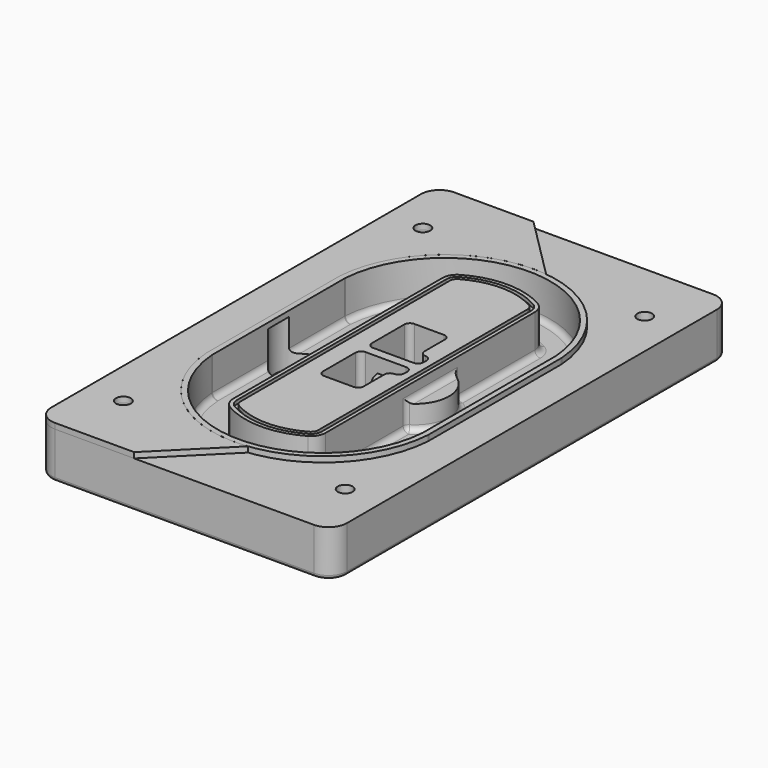
from build123d import *

# Parameters (mm, degrees)
F0_R      = 4
F1_DEPTH  = 25
F2_DEPTH  = 3
F3_DEPTH  = 18
F5_DEPTH  = 21
F6_DEPTH  = 2
F8_DEPTH  = 20
F9_DEPTH  = 16
F10_DEPTH = 25
F7_R      = 6
F7_R_2    = 4
F11_DEPTH = 6
F13_DEPTH = 9
F14_R     = 3
F15_R     = 2
F16_R     = 4
F17_DEPTH = 3


with BuildPart() as f1:
    # F0 (on Top) → F1 (new body)
    with BuildSketch(Plane.XY):
        with BuildLine():
            ThreePointArc((-80, -125), (-77.0710678119, -132.0710678119), (-70, -135))
            Line((-70, -135), (70, -135))
            ThreePointArc((70, -135), (77.0710678119, -132.0710678119), (80, -125))
            Line((80, -125), (80, 125))
            ThreePointArc((80, 125), (77.0710678119, 132.0710678119), (70, 135))
            Line((70, 135), (-70, 135))
            ThreePointArc((-70, 135), (-77.0710678119, 132.0710678119), (-80, 125))
            Line((-80, 125), (-80, -125))
        make_face()
        with Locations((-60, -101.25)):
            Circle(F0_R, mode=Mode.SUBTRACT)
        with Locations((60, -101.25)):
            Circle(F0_R, mode=Mode.SUBTRACT)
        with Locations((-60, 101.25)):
            Circle(F0_R, mode=Mode.SUBTRACT)
        with BuildLine():
            ThreePointArc((-64, 44.6627429245), (-63.991269098, 45.1571001106), (-63.9650872818, 45.650840699))
            ThreePointArc((-63.9650872818, 45.650840699), (0, 105.25), (63.9650872818, 45.650840699))
            ThreePointArc((63.9650872818, 45.650840699), (63.991269098, 45.1571001106), (64, 44.6627429245))
            Line((64, 44.6627429245), (64, -44.6627429245))
            ThreePointArc((64, -44.6627429245), (63.991269098, -45.1571001106), (63.9650872818, -45.650840699))
            ThreePointArc((63.9650872818, -45.650840699), (0, -105.25), (-63.9650872818, -45.650840699))
            ThreePointArc((-63.9650872818, -45.650840699), (-63.991269098, -45.1571001106), (-64, -44.6627429245))
            Line((-64, -44.6627429245), (-64, 44.6627429245))
        make_face(mode=Mode.SUBTRACT)
        with Locations((60, 101.25)):
            Circle(F0_R, mode=Mode.SUBTRACT)
        with BuildLine():
            ThreePointArc((63.9650872818, 45.650840699), (0, 105.25), (-63.9650872818, 45.650840699))
            ThreePointArc((-63.9650872818, 45.650840699), (-63.991269098, 45.1571001106), (-64, 44.6627429245))
            Line((-64, 44.6627429245), (-64, -44.6627429245))
            ThreePointArc((-64, -44.6627429245), (-63.991269098, -45.1571001106), (-63.9650872818, -45.650840699))
            ThreePointArc((-63.9650872818, -45.650840699), (0, -105.25), (63.9650872818, -45.650840699))
            ThreePointArc((63.9650872818, -45.650840699), (63.991269098, -45.1571001106), (64, -44.6627429245))
            Line((64, -44.6627429245), (64, 44.6627429245))
            ThreePointArc((64, 44.6627429245), (63.991269098, 45.1571001106), (63.9650872818, 45.650840699))
        make_face()
        with BuildLine():
            Line((-60, -44.6627429245), (-60, 44.6627429245))
            ThreePointArc((-60, 44.6627429245), (-59.9937636414, 45.0158552003), (-59.9750623441, 45.3685270491))
            ThreePointArc((-59.9750623441, 45.3685270491), (0, 101.25), (59.9750623441, 45.3685270491))
            ThreePointArc((59.9750623441, 45.3685270491), (59.9937636414, 45.0158552003), (60, 44.6627429245))
            Line((60, 44.6627429245), (60, -44.6627429245))
            ThreePointArc((60, -44.6627429245), (59.9937636414, -45.0158552003), (59.9750623441, -45.3685270491))
            ThreePointArc((59.9750623441, -45.3685270491), (0, -101.25), (-59.9750623441, -45.3685270491))
            ThreePointArc((-59.9750623441, -45.3685270491), (-59.9937636414, -45.0158552003), (-60, -44.6627429245))
        make_face(mode=Mode.SUBTRACT)
        with BuildLine():
            ThreePointArc((-59.9750623441, 45.3685270491), (-59.9937636414, 45.0158552003), (-60, 44.6627429245))
            Line((-60, 44.6627429245), (-60, -44.6627429245))
            ThreePointArc((-60, -44.6627429245), (-59.9937636414, -45.0158552003), (-59.9750623441, -45.3685270491))
            ThreePointArc((-59.9750623441, -45.3685270491), (0, -101.25), (59.9750623441, -45.3685270491))
            ThreePointArc((59.9750623441, -45.3685270491), (59.9937636414, -45.0158552003), (60, -44.6627429245))
            Line((60, -44.6627429245), (60, 44.6627429245))
            ThreePointArc((60, 44.6627429245), (59.9937636414, 45.0158552003), (59.9750623441, 45.3685270491))
            ThreePointArc((59.9750623441, 45.3685270491), (0, 101.25), (-59.9750623441, 45.3685270491))
        make_face()
        with BuildLine():
            ThreePointArc((56.9825436409, 45.1567918117), (56.995634549, 44.9099215176), (57, 44.6627429245))
            Line((57, 44.6627429245), (57, -44.6627429245))
            ThreePointArc((57, -44.6627429245), (56.995634549, -44.9099215176), (56.9825436409, -45.1567918117))
            ThreePointArc((56.9825436409, -45.1567918117), (0, -98.25), (-56.9825436409, -45.1567918117))
            ThreePointArc((-56.9825436409, -45.1567918117), (-56.995634549, -44.9099215176), (-57, -44.6627429245))
            Line((-57, -44.6627429245), (-57, 44.6627429245))
            ThreePointArc((-57, 44.6627429245), (-56.995634549, 44.9099215176), (-56.9825436409, 45.1567918117))
            ThreePointArc((-56.9825436409, 45.1567918117), (0, 98.25), (56.9825436409, 45.1567918117))
        make_face(mode=Mode.SUBTRACT)
        with BuildLine():
            Line((57, -44.6627429245), (57, 44.6627429245))
            ThreePointArc((57, 44.6627429245), (56.995634549, 44.9099215176), (56.9825436409, 45.1567918117))
            ThreePointArc((56.9825436409, 45.1567918117), (0, 98.25), (-56.9825436409, 45.1567918117))
            ThreePointArc((-56.9825436409, 45.1567918117), (-56.995634549, 44.9099215176), (-57, 44.6627429245))
            Line((-57, 44.6627429245), (-57, -44.6627429245))
            ThreePointArc((-57, -44.6627429245), (-56.995634549, -44.9099215176), (-56.9825436409, -45.1567918117))
            ThreePointArc((-56.9825436409, -45.1567918117), (0, -98.25), (56.9825436409, -45.1567918117))
            ThreePointArc((56.9825436409, -45.1567918117), (56.995634549, -44.9099215176), (57, -44.6627429245))
        make_face()
    extrude(amount=-F1_DEPTH)

    # F0 (on Top) → F2 (join)
    with BuildSketch(Plane.XY):
        with BuildLine():
            ThreePointArc((-59.9750623441, 45.3685270491), (-59.9937636414, 45.0158552003), (-60, 44.6627429245))
            Line((-60, 44.6627429245), (-60, -44.6627429245))
            ThreePointArc((-60, -44.6627429245), (-59.9937636414, -45.0158552003), (-59.9750623441, -45.3685270491))
            ThreePointArc((-59.9750623441, -45.3685270491), (0, -101.25), (59.9750623441, -45.3685270491))
            ThreePointArc((59.9750623441, -45.3685270491), (59.9937636414, -45.0158552003), (60, -44.6627429245))
            Line((60, -44.6627429245), (60, 44.6627429245))
            ThreePointArc((60, 44.6627429245), (59.9937636414, 45.0158552003), (59.9750623441, 45.3685270491))
            ThreePointArc((59.9750623441, 45.3685270491), (0, 101.25), (-59.9750623441, 45.3685270491))
        make_face()
        with BuildLine():
            ThreePointArc((56.9825436409, 45.1567918117), (56.995634549, 44.9099215176), (57, 44.6627429245))
            Line((57, 44.6627429245), (57, -44.6627429245))
            ThreePointArc((57, -44.6627429245), (56.995634549, -44.9099215176), (56.9825436409, -45.1567918117))
            ThreePointArc((56.9825436409, -45.1567918117), (0, -98.25), (-56.9825436409, -45.1567918117))
            ThreePointArc((-56.9825436409, -45.1567918117), (-56.995634549, -44.9099215176), (-57, -44.6627429245))
            Line((-57, -44.6627429245), (-57, 44.6627429245))
            ThreePointArc((-57, 44.6627429245), (-56.995634549, 44.9099215176), (-56.9825436409, 45.1567918117))
            ThreePointArc((-56.9825436409, 45.1567918117), (0, 98.25), (56.9825436409, 45.1567918117))
        make_face(mode=Mode.SUBTRACT)
    extrude(amount=F2_DEPTH)

    # F0 (on Top) → F3 (cut)
    with BuildSketch(Plane.XY):
        with BuildLine():
            Line((57, -44.6627429245), (57, 44.6627429245))
            ThreePointArc((57, 44.6627429245), (56.995634549, 44.9099215176), (56.9825436409, 45.1567918117))
            ThreePointArc((56.9825436409, 45.1567918117), (0, 98.25), (-56.9825436409, 45.1567918117))
            ThreePointArc((-56.9825436409, 45.1567918117), (-56.995634549, 44.9099215176), (-57, 44.6627429245))
            Line((-57, 44.6627429245), (-57, -44.6627429245))
            ThreePointArc((-57, -44.6627429245), (-56.995634549, -44.9099215176), (-56.9825436409, -45.1567918117))
            ThreePointArc((-56.9825436409, -45.1567918117), (0, -98.25), (56.9825436409, -45.1567918117))
            ThreePointArc((56.9825436409, -45.1567918117), (56.995634549, -44.9099215176), (57, -44.6627429245))
        make_face()
    extrude(amount=-F3_DEPTH, mode=Mode.SUBTRACT)

    # F4 (on face) → F5 (join, through all)
    with BuildSketch(Plane.XY.offset(3)):
        with BuildLine():
            ThreePointArc((-25, -70.7141132851), (-23.9239722661, -74.7214325959), (-20.9853479853, -77.6507552274))
            ThreePointArc((-20.9853479853, -77.6507552274), (0, -83.25), (20.9853479853, -77.6507552274))
            ThreePointArc((20.9853479853, -77.6507552274), (23.9239722661, -74.7214325959), (25, -70.7141132851))
            Line((25, -70.7141132851), (25, 70.7141132851))
            ThreePointArc((25, 70.7141132851), (23.9239722661, 74.7214325959), (20.9853479853, 77.6507552274))
            ThreePointArc((20.9853479853, 77.6507552274), (0, 83.25), (-20.9853479853, 77.6507552274))
            ThreePointArc((-20.9853479853, 77.6507552274), (-23.9239722661, 74.7214325959), (-25, 70.7141132851))
            Line((-25, 70.7141132851), (-25, -70.7141132851))
        make_face()
        with BuildLine():
            ThreePointArc((19.989010989, 75.9165947419), (22.1929791996, 73.7196027682), (23, 70.7141132851))
            Line((23, 70.7141132851), (23, -70.7141132851))
            ThreePointArc((23, -70.7141132851), (22.1929791996, -73.7196027682), (19.989010989, -75.9165947419))
            ThreePointArc((19.989010989, -75.9165947419), (0, -81.25), (-19.989010989, -75.9165947419))
            ThreePointArc((-19.989010989, -75.9165947419), (-22.1929791996, -73.7196027682), (-23, -70.7141132851))
            Line((-23, -70.7141132851), (-23, 70.7141132851))
            ThreePointArc((-23, 70.7141132851), (-22.1929791996, 73.7196027682), (-19.989010989, 75.9165947419))
            ThreePointArc((-19.989010989, 75.9165947419), (0, 81.25), (19.989010989, 75.9165947419))
        make_face(mode=Mode.SUBTRACT)
        with BuildLine():
            Line((23, -70.7141132851), (23, 70.7141132851))
            ThreePointArc((23, 70.7141132851), (22.1929791996, 73.7196027682), (19.989010989, 75.9165947419))
            ThreePointArc((19.989010989, 75.9165947419), (0, 81.25), (-19.989010989, 75.9165947419))
            ThreePointArc((-19.989010989, 75.9165947419), (-22.1929791996, 73.7196027682), (-23, 70.7141132851))
            Line((-23, 70.7141132851), (-23, -70.7141132851))
            ThreePointArc((-23, -70.7141132851), (-22.1929791996, -73.7196027682), (-19.989010989, -75.9165947419))
            ThreePointArc((-19.989010989, -75.9165947419), (0, -81.25), (19.989010989, -75.9165947419))
            ThreePointArc((19.989010989, -75.9165947419), (22.1929791996, -73.7196027682), (23, -70.7141132851))
        make_face()
        with BuildLine():
            ThreePointArc((18.9926739927, 74.1824342563), (20.461986133, 72.7177729405), (21, 70.7141132851))
            Line((21, 70.7141132851), (21, -70.7141132851))
            ThreePointArc((21, -70.7141132851), (20.461986133, -72.7177729405), (18.9926739927, -74.1824342563))
            ThreePointArc((18.9926739927, -74.1824342563), (0, -79.25), (-18.9926739927, -74.1824342563))
            ThreePointArc((-18.9926739927, -74.1824342563), (-20.461986133, -72.7177729405), (-21, -70.7141132851))
            Line((-21, -70.7141132851), (-21, 70.7141132851))
            ThreePointArc((-21, 70.7141132851), (-20.461986133, 72.7177729405), (-18.9926739927, 74.1824342563))
            ThreePointArc((-18.9926739927, 74.1824342563), (0, 79.25), (18.9926739927, 74.1824342563))
        make_face(mode=Mode.SUBTRACT)
        with BuildLine():
            Line((21, -70.7141132851), (21, 70.7141132851))
            ThreePointArc((21, 70.7141132851), (20.461986133, 72.7177729405), (18.9926739927, 74.1824342563))
            ThreePointArc((18.9926739927, 74.1824342563), (0, 79.25), (-18.9926739927, 74.1824342563))
            ThreePointArc((-18.9926739927, 74.1824342563), (-20.461986133, 72.7177729405), (-21, 70.7141132851))
            Line((-21, 70.7141132851), (-21, -70.7141132851))
            ThreePointArc((-21, -70.7141132851), (-20.461986133, -72.7177729405), (-18.9926739927, -74.1824342563))
            ThreePointArc((-18.9926739927, -74.1824342563), (0, -79.25), (18.9926739927, -74.1824342563))
            ThreePointArc((18.9926739927, -74.1824342563), (20.461986133, -72.7177729405), (21, -70.7141132851))
        make_face()
        with BuildLine():
            Line((-8, -2.5), (14, -2.5))
            ThreePointArc((14, -2.5), (16.1213203436, -3.3786796564), (17, -5.5))
            Line((17, -5.5), (17, -7.5))
            ThreePointArc((17, -7.5), (16.1213203436, -9.6213203436), (14, -10.5))
            ThreePointArc((14, -10.5), (11.8786796564, -11.3786796564), (11, -13.5))
            Line((11, -13.5), (11, -27.5))
            ThreePointArc((11, -27.5), (10.1213203436, -29.6213203436), (8, -30.5))
            Line((8, -30.5), (-8, -30.5))
            ThreePointArc((-8, -30.5), (-10.1213203436, -29.6213203436), (-11, -27.5))
            Line((-11, -27.5), (-11, -5.5))
            ThreePointArc((-11, -5.5), (-10.1213203436, -3.3786796564), (-8, -2.5))
        make_face(mode=Mode.SUBTRACT)
        with BuildLine():
            ThreePointArc((-8, 2.5), (-10.1213203436, 3.3786796564), (-11, 5.5))
            Line((-11, 5.5), (-11, 27.5))
            ThreePointArc((-11, 27.5), (-10.1213203436, 29.6213203436), (-8, 30.5))
            Line((-8, 30.5), (8, 30.5))
            ThreePointArc((8, 30.5), (10.1213203436, 29.6213203436), (11, 27.5))
            Line((11, 27.5), (11, 13.5))
            ThreePointArc((11, 13.5), (11.8786796564, 11.3786796564), (14, 10.5))
            ThreePointArc((14, 10.5), (16.1213203436, 9.6213203436), (17, 7.5))
            Line((17, 7.5), (17, 5.5))
            ThreePointArc((17, 5.5), (16.1213203436, 3.3786796564), (14, 2.5))
            Line((14, 2.5), (-8, 2.5))
        make_face(mode=Mode.SUBTRACT)
    extrude(amount=-F5_DEPTH)

    # F4 (on face) → F6 (cut)
    with BuildSketch(Plane.XY.offset(3)):
        with BuildLine():
            Line((23, -70.7141132851), (23, 70.7141132851))
            ThreePointArc((23, 70.7141132851), (22.1929791996, 73.7196027682), (19.989010989, 75.9165947419))
            ThreePointArc((19.989010989, 75.9165947419), (0, 81.25), (-19.989010989, 75.9165947419))
            ThreePointArc((-19.989010989, 75.9165947419), (-22.1929791996, 73.7196027682), (-23, 70.7141132851))
            Line((-23, 70.7141132851), (-23, -70.7141132851))
            ThreePointArc((-23, -70.7141132851), (-22.1929791996, -73.7196027682), (-19.989010989, -75.9165947419))
            ThreePointArc((-19.989010989, -75.9165947419), (0, -81.25), (19.989010989, -75.9165947419))
            ThreePointArc((19.989010989, -75.9165947419), (22.1929791996, -73.7196027682), (23, -70.7141132851))
        make_face()
        with BuildLine():
            ThreePointArc((18.9926739927, 74.1824342563), (20.461986133, 72.7177729405), (21, 70.7141132851))
            Line((21, 70.7141132851), (21, -70.7141132851))
            ThreePointArc((21, -70.7141132851), (20.461986133, -72.7177729405), (18.9926739927, -74.1824342563))
            ThreePointArc((18.9926739927, -74.1824342563), (0, -79.25), (-18.9926739927, -74.1824342563))
            ThreePointArc((-18.9926739927, -74.1824342563), (-20.461986133, -72.7177729405), (-21, -70.7141132851))
            Line((-21, -70.7141132851), (-21, 70.7141132851))
            ThreePointArc((-21, 70.7141132851), (-20.461986133, 72.7177729405), (-18.9926739927, 74.1824342563))
            ThreePointArc((-18.9926739927, 74.1824342563), (0, 79.25), (18.9926739927, 74.1824342563))
        make_face(mode=Mode.SUBTRACT)
    extrude(amount=-F6_DEPTH, mode=Mode.SUBTRACT)

    # F7 (on face) → F8 (join)
    with BuildSketch(Plane(origin=(0, 0, -25), x_dir=(1, 0, 0), z_dir=(0, 0, -1))):
        with BuildLine():
            ThreePointArc((3.28842436, 0), (16.7567035675, 13.4682792075), (30.224982775, 0))
            Line((30.224982775, 0), (35.224982775, 0))
            ThreePointArc((35.224982775, 0), (16.7567035675, 18.4682792075), (-1.71157564, 0))
            Line((-1.71157564, 0), (3.28842436, 0))
        make_face()
        with BuildLine():
            Line((3.28842436, 0), (30.224982775, 0))
            ThreePointArc((30.224982775, 0), (16.7567035675, 13.4682792075), (3.28842436, 0))
        make_face()
        with BuildLine():
            ThreePointArc((3.28842436, 0), (16.7567035675, -13.4682792075), (30.224982775, 0))
            Line((30.224982775, 0), (3.28842436, 0))
        make_face()
        with BuildLine():
            Line((35.224982775, 0), (30.224982775, 0))
            ThreePointArc((30.224982775, 0), (16.7567035675, -13.4682792075), (3.28842436, 0))
            Line((3.28842436, 0), (-1.71157564, 0))
            ThreePointArc((-1.71157564, 0), (16.7567035675, -18.4682792075), (35.224982775, 0))
        make_face()
    extrude(amount=-F8_DEPTH)

    # F7 (on face) → F9 (cut)
    with BuildSketch(Plane(origin=(0, 0, -25), x_dir=(1, 0, 0), z_dir=(0, 0, -1))):
        with BuildLine():
            Line((3.28842436, 0), (30.224982775, 0))
            ThreePointArc((30.224982775, 0), (16.7567035675, 13.4682792075), (3.28842436, 0))
        make_face()
        with BuildLine():
            ThreePointArc((3.28842436, 0), (16.7567035675, -13.4682792075), (30.224982775, 0))
            Line((30.224982775, 0), (3.28842436, 0))
        make_face()
    extrude(amount=-F9_DEPTH, mode=Mode.SUBTRACT)

    # F7 (on face) → F10 (cut)
    with BuildSketch(Plane(origin=(0, 0, -25), x_dir=(1, 0, 0), z_dir=(0, 0, -1))):
        with BuildLine():
            Line((-59.0318229325, 0), (-32.0952645175, 0))
            ThreePointArc((-32.0952645175, 0), (-45.563543725, 13.4682792075), (-59.0318229325, 0))
        make_face()
        with BuildLine():
            ThreePointArc((-59.0318229325, 0), (-45.563543725, -13.4682792075), (-32.0952645175, 0))
            Line((-32.0952645175, 0), (-59.0318229325, 0))
        make_face()
    extrude(amount=-F10_DEPTH, mode=Mode.SUBTRACT)

    # F7 (on face) → F11 (cut)
    with BuildSketch(Plane(origin=(0, 0, -25), x_dir=(1, 0, 0), z_dir=(0, 0, -1))):
        with Locations((60, -101.25)):
            Circle(F7_R)
        with Locations((60, -101.25)):
            Circle(F7_R_2, mode=Mode.SUBTRACT)
        with Locations((-60, -101.25)):
            Circle(F7_R)
        with Locations((-60, -101.25)):
            Circle(F7_R_2, mode=Mode.SUBTRACT)
        with Locations((-60, 101.25)):
            Circle(F7_R)
        with Locations((-60, 101.25)):
            Circle(F7_R_2, mode=Mode.SUBTRACT)
        with Locations((60, 101.25)):
            Circle(F7_R)
        with Locations((60, 101.25)):
            Circle(F7_R_2, mode=Mode.SUBTRACT)
    extrude(amount=-F11_DEPTH, mode=Mode.SUBTRACT)

    # F12 (on face) → F13 (cut, through all)
    with BuildSketch(Plane(origin=(0, 0, -9), x_dir=(1, 0, 0), z_dir=(0, 0, -1))):
        with BuildLine():
            Line((11, 13.5), (11, 17.5481537753))
            ThreePointArc((11, 17.5481537753), (2.5696536419, 11.8239143813), (-1.5415842455, 2.5))
            Line((-1.5415842455, 2.5), (3.5224848595, 2.5))
            ThreePointArc((3.5224848595, 2.5), (6.1857188154, 8.3455872281), (11.2536447004, 12.2927168648))
            ThreePointArc((11.2536447004, 12.2927168648), (11.0640958889, 12.8831798879), (11, 13.5))
        make_face()
        with BuildLine():
            ThreePointArc((11.2536447004, -12.2927168648), (6.1857188154, -8.3455872281), (3.5224848595, -2.5))
            Line((3.5224848595, -2.5), (-1.5415842455, -2.5))
            ThreePointArc((-1.5415842455, -2.5), (2.5696536419, -11.8239143813), (11, -17.5481537753))
            Line((11, -17.5481537753), (11, -13.5))
            ThreePointArc((11, -13.5), (11.0640958889, -12.8831798879), (11.2536447004, -12.2927168648))
        make_face()
        with BuildLine():
            ThreePointArc((11.2536447004, 12.2927168648), (6.1857188154, 8.3455872281), (3.5224848595, 2.5))
            Line((3.5224848595, 2.5), (14, 2.5))
            ThreePointArc((14, 2.5), (16.1213203436, 3.3786796564), (17, 5.5))
            Line((17, 5.5), (17, 7.5))
            ThreePointArc((17, 7.5), (16.1213203436, 9.6213203436), (14, 10.5))
            ThreePointArc((14, 10.5), (12.3601599782, 10.9878446101), (11.2536447004, 12.2927168648))
        make_face()
        with BuildLine():
            Line((14, -2.5), (3.5224848595, -2.5))
            ThreePointArc((3.5224848595, -2.5), (6.1857188154, -8.3455872281), (11.2536447004, -12.2927168648))
            ThreePointArc((11.2536447004, -12.2927168648), (12.3601599782, -10.9878446101), (14, -10.5))
            ThreePointArc((14, -10.5), (16.1213203436, -9.6213203436), (17, -7.5))
            Line((17, -7.5), (17, -5.5))
            ThreePointArc((17, -5.5), (16.1213203436, -3.3786796564), (14, -2.5))
        make_face()
    extrude(amount=F13_DEPTH, mode=Mode.SUBTRACT)

    # F14
    f14_edges = [f1.edges().sort_by_distance(p)[0] for p in [
        (-57, -25.888126, -18),
        (-57, 25.888126, -18),
        (25, 0, -5),
        (25, 16.526506, -11.5),
        (25, -16.526506, -11.5),
        (25, -43.62031, -18),
        (35.224983, 0, -18),
        (25, 43.62031, -18),
        (0, -98.25, -18),
        (-56.995635, -44.909922, -18),
        (-56.995635, 44.909922, -18),
        (0, 98.25, -18),
        (56.995635, 44.909922, -18),
        (57, 0, -18),
        (56.995635, -44.909922, -18),
        (-25, 0, -18),
        (-23.923972, 74.721433, -18),
        (-23.923972, -74.721433, -18),
        (0, 83.25, -18),
        (0, -83.25, -18),
        (23.923972, 74.721433, -18),
        (23.923972, -74.721433, -18),
    ]]
    fillet(f14_edges, radius=F14_R)

    # F15
    f15_edges = [f1.edges().sort_by_distance(p)[0] for p in [
        (0, -135, -25),
        (-77.071068, -132.071068, -25),
        (-80, 0, -25),
        (-77.071068, 132.071068, -25),
        (77.071068, -132.071068, -25),
        (0, 135, -25),
        (80, 0, -25),
        (77.071068, 132.071068, -25),
    ]]
    fillet(f15_edges, radius=F15_R)


with BuildPart() as f17:
    # F16 (on face) → F17 (new body, through all)
    with BuildSketch(Plane.XY):
        with BuildLine():
            ThreePointArc((-59.9750623441, 45.3685270491), (-38.3455365451, 87.43520894), (7.0171973941, 100.839106924))
            Line((7.0171973941, 100.839106924), (-27.1436956819, 135))
            Line((-27.1436956819, 135), (-70, 135))
            ThreePointArc((-70, 135), (-77.0710678119, 132.0710678119), (-80, 125))
            Line((-80, 125), (-80, -125))
            ThreePointArc((-80, -125), (-77.0710678119, -132.0710678119), (-70, -135))
            Line((-70, -135), (-27.1436956819, -135))
            Line((-27.1436956819, -135), (7.0171973941, -100.839106924))
            ThreePointArc((7.0171973941, -100.839106924), (-38.3455365451, -87.43520894), (-59.9750623441, -45.3685270491))
            ThreePointArc((-59.9750623441, -45.3685270491), (-59.9937636414, -45.0158552003), (-60, -44.6627429245))
            Line((-60, -44.6627429245), (-60, 44.6627429245))
            ThreePointArc((-60, 44.6627429245), (-59.9937636414, 45.0158552003), (-59.9750623441, 45.3685270491))
        make_face()
        with Locations((-60, -101.25)):
            Circle(F16_R, mode=Mode.SUBTRACT)
        with Locations((-60, 101.25)):
            Circle(F16_R, mode=Mode.SUBTRACT)
    extrude(amount=F17_DEPTH)


solid = Compound([f1.part, f17.part])
